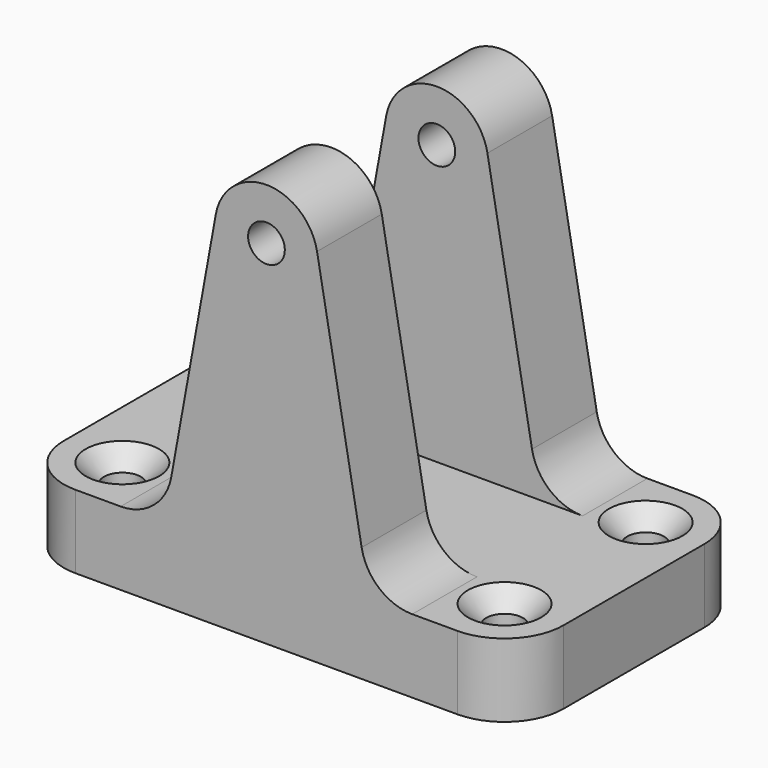
from build123d import *

# Parameters (mm, degrees)
F0_R      = 2.5
F1_DEPTH  = 40
F2_R      = 5
F2_R_2    = 2.5
F3_DEPTH  = 3
F4_W      = 32.6441857368
F4_H      = 17.9751312453
F5_DEPTH  = 50
F6_R      = 8
F9_R      = 7
F7_R      = 5
F7_R_2    = 2.5
F10_DEPTH = 3
F11_DEPTH = 25
F12_SIZE2 = 2.5
F12_SIZE  = 2.5


with BuildPart() as f1:
    # F0 (on Front) → F1 (new body)
    with BuildSketch(Plane.XZ):
        with BuildLine():
            Line((-6.8878248776, 9.4542597632), (-14, -29.7938862443))
            Line((-14, -29.7938862443), (14, -29.7938862443))
            Line((14, -29.7938862443), (6.8878248776, 9.4542597632))
            ThreePointArc((6.8878248776, 9.4542597632), (0, 15.2061137557), (-6.8878248776, 9.4542597632))
        make_face()
        with Locations((0, 8.2061137557)):
            Circle(F0_R, mode=Mode.SUBTRACT)
        Polygon((-34, -39.7938862443), (0, -39.7938862443), (34, -39.7938862443), (34, -29.7938862443), (14, -29.7938862443), (-14, -29.7938862443), (-34, -29.7938862443), align=None)
    extrude(amount=-F1_DEPTH)

    # F2 (on face) → F3 (cut)
    with BuildSketch(Plane.XY.offset(-29.7938862443)):
        with Locations((26.0093560517, 32)):
            Circle(F2_R)
        with Locations((26.0093560517, 32)):
            Circle(F2_R_2, mode=Mode.SUBTRACT)
        with Locations((-26.0093560517, 32)):
            Circle(F2_R)
        with Locations((-26.0093560517, 32)):
            Circle(F2_R_2, mode=Mode.SUBTRACT)
        with Locations((-26.0093560517, 8)):
            Circle(F2_R)
        with Locations((-26.0093560517, 8)):
            Circle(F2_R_2, mode=Mode.SUBTRACT)
        with Locations((26.0093560517, 8)):
            Circle(F2_R)
        with Locations((26.0093560517, 8)):
            Circle(F2_R_2, mode=Mode.SUBTRACT)
    extrude(amount=-F3_DEPTH, mode=Mode.SUBTRACT)

    # F4 (on face) → F5 (cut)
    with BuildSketch(Plane.XY.offset(-29.7938862443)):
        with Locations((2.3220928684, 20)):
            Rectangle(F4_W, F4_H)
    extrude(amount=F5_DEPTH, mode=Mode.SUBTRACT)

    # F6
    f6_edges = [f1.edges().sort_by_distance(p)[0] for p in [
        (-34, 0, -34.793886),
        (34, 0, -34.793886),
        (34, 40, -34.793886),
        (-34, 40, -34.793886),
    ]]
    fillet(f6_edges, radius=F6_R)

    # F9
    f9_edges = [f1.edges().sort_by_distance(p)[0] for p in [
        (-14, 5.506217, -29.793886),
        (-14, 34.493783, -29.793886),
        (14, 5.506217, -29.793886),
        (14, 34.493783, -29.793886),
    ]]
    fillet(f9_edges, radius=F9_R)

    # F7 (on face) → F10 (join)
    with BuildSketch(Plane.XY.offset(-32.7938862443)):
        with Locations((-26.0093560517, 32)):
            Circle(F7_R)
        with Locations((-26.0093560517, 32)):
            Circle(F7_R_2, mode=Mode.SUBTRACT)
        with Locations((26.0093560517, 32)):
            Circle(F7_R)
        with Locations((26.0093560517, 32)):
            Circle(F7_R_2, mode=Mode.SUBTRACT)
        with Locations((26.0093560517, 8)):
            Circle(F7_R)
        with Locations((26.0093560517, 8)):
            Circle(F7_R_2, mode=Mode.SUBTRACT)
        with Locations((-26.0093560517, 8)):
            Circle(F7_R)
        with Locations((-26.0093560517, 8)):
            Circle(F7_R_2, mode=Mode.SUBTRACT)
    extrude(amount=F10_DEPTH)

    # F2 (on face) → F11 (cut)
    with BuildSketch(Plane.XY.offset(-29.7938862443)):
        with Locations((-26.0093560517, 32)):
            Circle(F2_R_2)
        with Locations((-26.0093560517, 8)):
            Circle(F2_R_2)
        with Locations((26.0093560517, 8)):
            Circle(F2_R_2)
        with Locations((26.0093560517, 32)):
            Circle(F2_R_2)
    extrude(amount=-F11_DEPTH, mode=Mode.SUBTRACT)

    # F12
    f12_edges = [f1.edges().sort_by_distance(p)[0] for p in [
        (-28.509356, 32, -29.793886),
        (23.509356, 32, -29.793886),
        (23.509356, 8, -29.793886),
        (-28.509356, 8, -29.793886),
    ]]
    chamfer(f12_edges, length=F12_SIZE, length2=F12_SIZE2)


solid = f1.part
